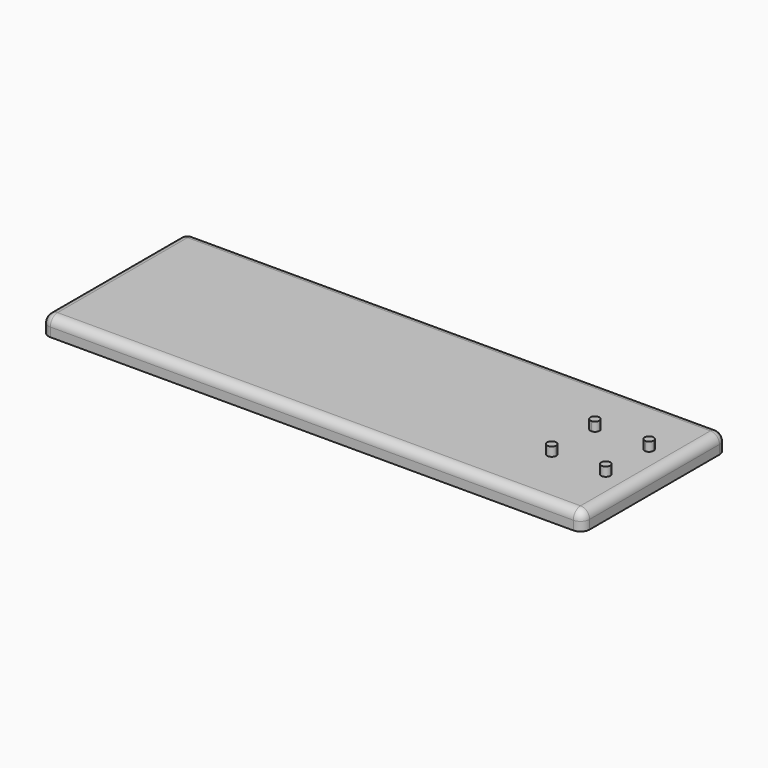
from build123d import *

# Parameters (mm, degrees)
F0_W     = 762
F0_H     = 254
F1_DEPTH = 25.4
F3_R     = 12.7
F5_DEPTH = 12.7


# Not quite as in the source:
# - a feature of the source that left no trace in its solid (it failed there, or was rolled back) is left out


with BuildPart() as f1:
    # F0 (on Top) → F1 (new body)
    with BuildSketch(Plane.XY):
        with Locations((-381, -127)):
            Rectangle(F0_W, F0_H)
    extrude(amount=F1_DEPTH)

    # F3
    f3_edges = [f1.edges().sort_by_distance(p)[0] for p in [
        (-762, -254, 12.7),
        (0, -254, 12.7),
        (0, 0, 12.7),
        (0, -127, 25.4),
        (-762, 0, 12.7),
        (-381, 0, 25.4),
        (-762, -127, 25.4),
        (-381, -254, 25.4),
    ]]
    fillet(f3_edges, radius=F3_R)

    # F4 (on face) → F5 (join)
    with BuildSketch(Plane.XY.offset(25.4)):
        with BuildLine():
            Line((-44.45, -165.1), (-38.1, -165.1))
            Line((-38.1, -165.1), (-38.1, -158.75))
            ThreePointArc((-38.1, -158.75), (-42.5901280605, -160.6098719395), (-44.45, -165.1))
        make_face()
        with BuildLine():
            ThreePointArc((-44.45, -165.1), (-38.1, -171.45), (-31.75, -165.1))
            Line((-31.75, -165.1), (-38.1, -165.1))
            Line((-38.1, -165.1), (-44.45, -165.1))
        make_face()
        with BuildLine():
            Line((-38.1, -165.1), (-31.75, -165.1))
            ThreePointArc((-31.75, -165.1), (-33.6098719395, -160.6098719395), (-38.1, -158.75))
            Line((-38.1, -158.75), (-38.1, -165.1))
        make_face()
        with BuildLine():
            Line((-114.3, -165.1), (-107.95, -165.1))
            ThreePointArc((-107.95, -165.1), (-109.8098719395, -160.6098719395), (-114.3, -158.75))
            Line((-114.3, -158.75), (-114.3, -165.1))
        make_face()
        with BuildLine():
            ThreePointArc((-114.3, -158.75), (-118.7901280605, -169.5901280605), (-107.95, -165.1))
            Line((-107.95, -165.1), (-114.3, -165.1))
            Line((-114.3, -165.1), (-114.3, -158.75))
        make_face()
        with BuildLine():
            ThreePointArc((-114.3, -95.25), (-109.8098719395, -93.3901280605), (-107.95, -88.9))
            Line((-107.95, -88.9), (-114.3, -88.9))
            Line((-114.3, -88.9), (-114.3, -95.25))
        make_face()
        with BuildLine():
            Line((-114.3, -88.9), (-107.95, -88.9))
            ThreePointArc((-107.95, -88.9), (-118.7901280605, -84.4098719395), (-114.3, -95.25))
            Line((-114.3, -95.25), (-114.3, -88.9))
        make_face()
        with BuildLine():
            Line((-38.1, -88.9), (-31.75, -88.9))
            ThreePointArc((-31.75, -88.9), (-38.1, -82.55), (-44.45, -88.9))
            Line((-44.45, -88.9), (-38.1, -88.9))
        make_face()
        with BuildLine():
            Line((-38.1, -95.25), (-38.1, -88.9))
            Line((-38.1, -88.9), (-44.45, -88.9))
            ThreePointArc((-44.45, -88.9), (-42.5901280605, -93.3901280605), (-38.1, -95.25))
        make_face()
        with BuildLine():
            ThreePointArc((-38.1, -95.25), (-33.6098719395, -93.3901280605), (-31.75, -88.9))
            Line((-31.75, -88.9), (-38.1, -88.9))
            Line((-38.1, -88.9), (-38.1, -95.25))
        make_face()
    extrude(amount=F5_DEPTH)


solid = f1.part
